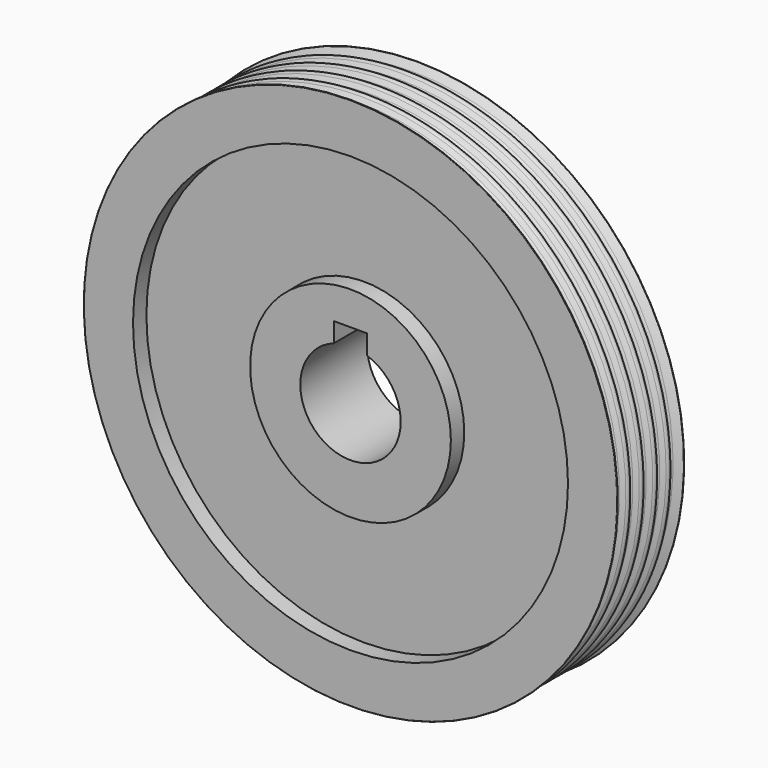
from build123d import *

# Parameters (mm, degrees)
F0_R     = 101.6
F0_R_2   = 19.05
F1_DEPTH = 31.75
F2_R     = 82.55
F2_R_2   = 38.1
F3_DEPTH = 6.35
F4_R     = 82.55
F4_R_2   = 38.1
F5_DEPTH = 6.35
F6_W     = 12.7
F6_H     = 12.7
F7_DEPTH = 31.751
F10_R    = 0.127
F11_R    = 1.27


with BuildPart() as f1:
    # F0 (on Front) → F1 (new body)
    with BuildSketch(Plane.XZ):
        Circle(F0_R)
        Circle(F0_R_2, mode=Mode.SUBTRACT)
    extrude(amount=F1_DEPTH)

    # F2 (on face) → F3 (cut)
    with BuildSketch(Plane.XZ.offset(31.75)):
        Circle(F2_R)
        Circle(F2_R_2, mode=Mode.SUBTRACT)
    extrude(amount=-F3_DEPTH, mode=Mode.SUBTRACT)

    # F4 (on face) → F5 (cut)
    with BuildSketch(Plane(origin=(0, 0, 0), x_dir=(-1, 0, 0), z_dir=(0, 1, 0))):
        Circle(F4_R)
        Circle(F4_R_2, mode=Mode.SUBTRACT)
    extrude(amount=-F5_DEPTH, mode=Mode.SUBTRACT)

    # F6 (on face) → F7 (cut, through all)
    with BuildSketch(Plane.XZ.offset(31.75)):
        with Locations((0, 19.05)):
            Rectangle(F6_W, F6_H)
    extrude(amount=-F7_DEPTH, mode=Mode.SUBTRACT)

    # F8 (on Right) → F9 (revolve, cut)
    with BuildSketch(Plane.YZ):
        Polygon((-3.175, 97.4581763148), (0, 101.5856489539), (0, 113.58909374), (-31.7767225206, 113.58909374), (-31.7767225206, 101.5856489539), (-28.6017225206, 97.4581763148), (-25.4267225206, 101.5856489539), (-22.2517225206, 97.4581763148), (-19.0767225206, 101.5856489539), (-15.9017225206, 97.4581763148), (-12.7, 101.5856489539), (-9.525, 97.4581763148), (-6.35, 101.5856489539), align=None)
    revolve(axis=Axis((0, 0, 0), (0, 1, 0)), mode=Mode.SUBTRACT)

    # F10
    f10_edges = [f1.edges().sort_by_distance(p)[0] for p in [
        (0, 0, -101.585649),
        (0, -31.75, -101.55091),
    ]]
    fillet(f10_edges, radius=F10_R)

    # F11
    f11_edges = [f1.edges().sort_by_distance(p)[0] for p in [
        (0, -3.175, -97.458176),
        (0, -9.525, -97.458176),
        (0, -15.901723, -97.458176),
        (0, -22.251723, -97.458176),
        (0, -28.601723, -97.458176),
        (0, -25.426723, -101.585649),
        (0, -19.076723, -101.585649),
        (0, -12.7, -101.585649),
        (0, -6.35, -101.585649),
    ]]
    fillet(f11_edges, radius=F11_R)


solid = f1.part
